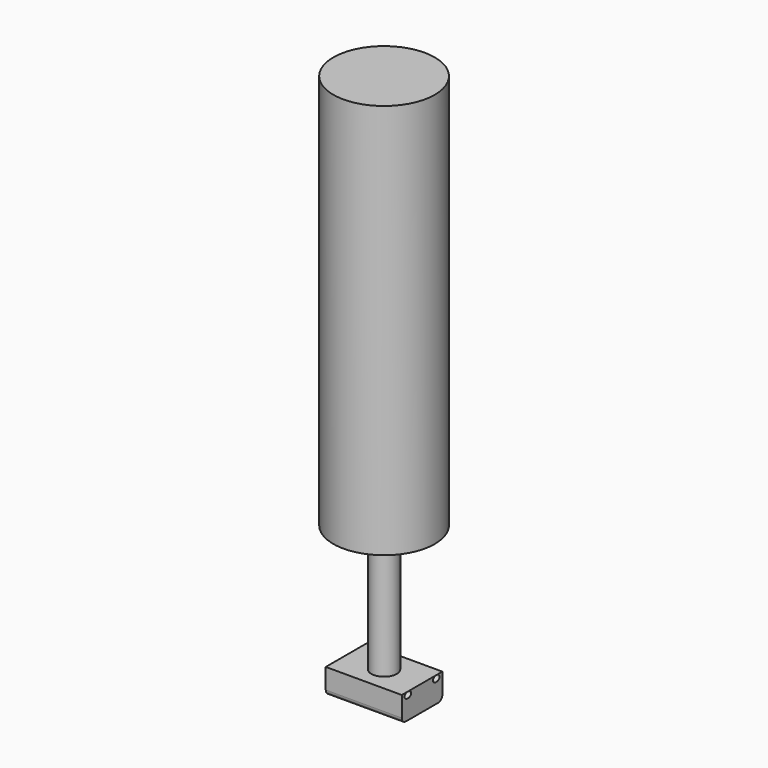
from build123d import *

# Parameters (mm, degrees)
F0_W      = 15
F0_H      = 10
F1_DEPTH  = 5
F2_R      = 2.5
F3_DEPTH  = 100
F6_R      = 1
F9_DEPTH  = 15.001
F5_R      = 10
F10_DEPTH = 75
F11_R     = 8
F12_DEPTH = 72
F13_R     = 10
F13_R_2   = 8
F15_DEPTH = 3


with BuildPart() as f1:
    # F0 (on Top) → F1 (new body)
    with BuildSketch(Plane.XY):
        with Locations((7.5, 5)):
            Rectangle(F0_W, F0_H)
    extrude(amount=F1_DEPTH)

    # F2 (on face) → F3 (join)
    with BuildSketch(Plane.XY.offset(5)):
        with Locations((7.5, 5)):
            Circle(F2_R)
    extrude(amount=F3_DEPTH)

    # F6
    f6_edges = [f1.edges().sort_by_distance(p)[0] for p in [
        (7.5, 0, 0),
        (7.5, 10, 0),
    ]]
    fillet(f6_edges, radius=F6_R)

    # F7 (on face) → F9 (cut, through all)
    with BuildSketch(Plane.YZ.offset(15)):
        with BuildLine():
            add(Edge.make_bspline(
                [(1.5, 4.9999053105), (-0.491726189, 4.9999053105), (0.9166369055, 3.9758028869), (2.325, 2.9517004633), (2.325, 4.4)],
                knots=[1.5707963268, 1.5707963268, 1.5707963268, 3.926990817, 3.926990817, 6.2831853072, 6.2831853072, 6.2831853072], degree=2, weights=[1, 0.3826834324, 1, 0.3826834324, 1]))
            add(Edge.make_bspline(
                [(2.325, 4.4), (2.325, 4.9999053105), (1.5, 4.9999053105)],
                knots=[0, 0, 0, 1.5707963268, 1.5707963268, 1.5707963268], degree=2, weights=[1, 0.7071067812, 1]))
        make_face()
        with BuildLine():
            add(Edge.make_bspline(
                [(7.675, 4.4), (7.675, 2.9517004633), (9.0833630945, 3.9758028869), (10.491726189, 4.9999053105), (8.5, 4.9999053105)],
                knots=[0, 0, 0, 2.3561944902, 2.3561944902, 4.7123889804, 4.7123889804, 4.7123889804], degree=2, weights=[1, 0.3826834324, 1, 0.3826834324, 1]))
            add(Edge.make_bspline(
                [(8.5, 4.9999053105), (7.675, 4.9999053105), (7.675, 4.4)],
                knots=[4.7123889804, 4.7123889804, 4.7123889804, 6.2831853072, 6.2831853072, 6.2831853072], degree=2, weights=[1, 0.7071067812, 1]))
        make_face()
    extrude(amount=-F9_DEPTH, mode=Mode.SUBTRACT)

    # F5 (on offset) → F10 (join, through all)
    with BuildSketch(Plane.XY.offset(30)):
        with Locations((7.5, 5)):
            Circle(F5_R)
    extrude(amount=F10_DEPTH)

    # F11 (on face) → F12 (cut)
    with BuildSketch(Plane.XY.offset(105)):
        with Locations((7.5, 5)):
            Circle(F11_R)
    extrude(amount=-F12_DEPTH, mode=Mode.SUBTRACT)

    # F13 (on face) → F15 (join)
    with BuildSketch(Plane.XY.offset(105)):
        with Locations((7.5, 5)):
            Circle(F13_R)
        with Locations((7.5, 5)):
            Circle(F13_R_2, mode=Mode.SUBTRACT)
        with Locations((7.5, 5)):
            Circle(F13_R_2)
    extrude(amount=F15_DEPTH)


solid = f1.part
